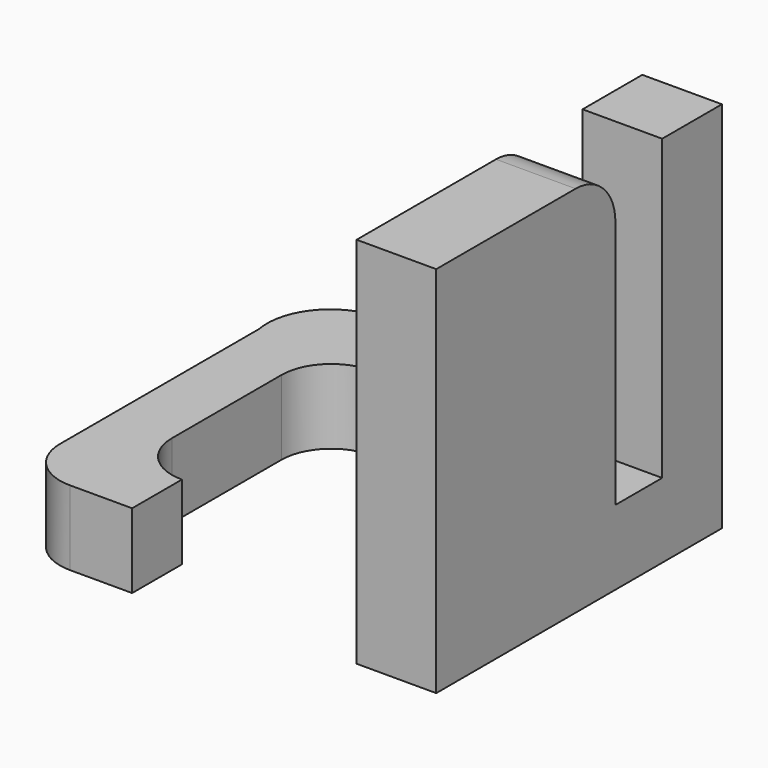
from build123d import *

# Parameters (mm, degrees)
F0_W        = 3.2
F0_H        = 9
F1_DEPTH    = 15
F0_H_2      = 3
F0_H_3      = 2.35
F2_DEPTH    = 3
F3_R        = 2
F4_R        = 1.99999
F5_T1_DEPTH = 3


# Not quite as in the source:
# - a fillet or chamfer that OpenCascade refuses, or shapes differently, is made with other operations: its cross-section is extruded or revolved along the edge and cut away or added
# - a fillet or chamfer is up to 0.001 mm smaller than in the source, because OpenCascade refuses the exact size


with BuildPart() as f1:
    # F0 (on Top) → F1 (new body)
    with BuildSketch(Plane.XY):
        with Locations((-1.6, 4.5)):
            Rectangle(F0_W, F0_H)
    extrude(amount=F1_DEPTH)



with BuildPart() as f1b:
    # F0 (on Top) → F1, piece 2 (new body)
    with BuildSketch(Plane.XY):
        with Locations((-1.6, 12.85)):
            Rectangle(F0_W, F0_H_2)
    extrude(amount=F1_DEPTH)


with BuildPart() as f1_1:
    add(f1.part)

    add(f1b.part)  # F2 merges F1b
    # F0 (on Top) → F2 (join)
    with BuildSketch(Plane.XY):
        with Locations((-1.6, 10.175)):
            Rectangle(F0_W, F0_H_3)
        with BuildLine():
            Line((-13.7, 11.35), (-3.2, 11.35))
            Line((-3.2, 11.35), (-3.2, 14.35))
            Line((-3.2, 14.35), (-13.7, 14.35))
            ThreePointArc((-13.7, 14.35), (-15.652562419, 13.4354686825), (-16.2, 11.35))
            Line((-16.2, 11.35), (-16.2, -0.65))
            Line((-16.2, -0.65), (-13.7, -0.65))
            Line((-13.7, -0.65), (-11.7, -0.65))
            Line((-11.7, -0.65), (-11.7, 1.85))
            Line((-11.7, 1.85), (-13.7, 1.85))
            Line((-13.7, 1.85), (-13.7, 11.35))
        make_face()
    extrude(amount=F2_DEPTH)

    # F3
    f3_edges = [f1_1.edges().sort_by_distance(p)[0] for p in [
        (-1.6, 9, 15),
    ]]
    fillet(f3_edges, radius=F3_R)

    # F4 (radius 2 in the source; OpenCascade refuses exactly that, so slightly less here)
    f4_edges = [f1_1.edges().sort_by_distance(p)[0] for p in [
        (-16.2, -0.65, 1.5),
        (-13.7, 11.35, 1.5),
        (-13.7, 1.85, 1.5),
    ]]
    fillet(f4_edges, radius=F4_R)

    # F5: fillet of radius 5 on 1 edges, made by hand

    # F5_s2 → F5_t1 (join)
    with BuildSketch(Plane.XZ.offset(-14.35)):
        with BuildLine():
            ThreePointArc((-8.2, 3), (-4.6644660941, 4.4644660941), (-3.2, 8))
            Line((-3.2, 8), (-3.2, 3))
            Line((-3.2, 3), (-8.2, 3))
        make_face()
    extrude(amount=F5_T1_DEPTH)


solid = f1_1.part
